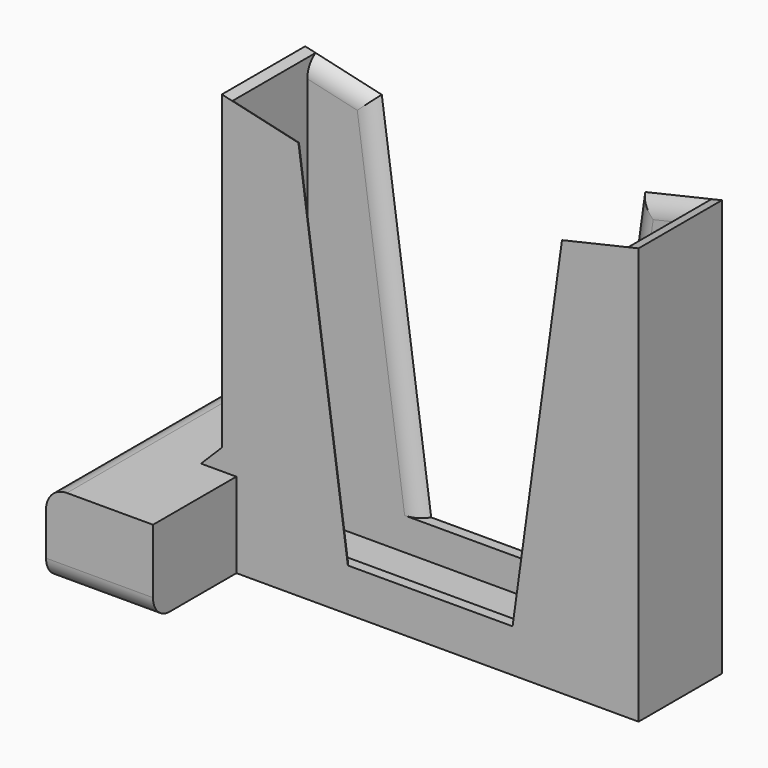
from build123d import *

# Parameters (mm, degrees)
F1_DEPTH     = 25.4
F2_T         = -2.54
F3_T4_DEPTH  = 109.6353324848
F3_T9_DEPTH  = 109.6353324848
F3_T14_DEPTH = 38.5537016023
F3_T19_DEPTH = 38.5537016023
F3_T24_DEPTH = 109.6353324848
F3_T29_DEPTH = 38.5537016023
F3_T34_DEPTH = 109.6353324848
F3_T39_DEPTH = 38.5537016023
F4_W         = 7.5721852481
F4_H         = 7.5721852481
F5_DEPTH     = 50.8
F6_SIZE      = 5.08
F7_R         = 5.08


# Not quite as in the source:
# - a fillet or chamfer that OpenCascade refuses, or shapes differently, is made with other operations: its cross-section is extruded or revolved along the edge and cut away or added


with BuildPart() as f1:
    # F0 (on Front) → F1 (new body)
    with BuildSketch(Plane.XZ):
        Polygon((-50.8, -50.8), (50.8, -50.8), (50.8, 50.8), (32.1275666356, 46.4897789061), (20.0797300786, -40.3164364398), (-20.0797300786, -40.3164364398), (-32.1275666356, 46.4897789061), (-50.8, 50.8), align=None)
    extrude(amount=F1_DEPTH)

    # F2
    f2_openings = [f1.faces().sort_by_distance(p)[0] for p in [
        (-41.463783, -12.7, 48.644889),
        (-26.103648, -12.7, 3.086671),
        (0, -12.7, -40.316436),
        (41.463783, -12.7, 48.644889),
        (26.103648, -12.7, 3.086671),
    ]]
    offset(amount=F2_T, openings=f2_openings)

    # F3: fillet of radius 5.08 on 8 edges, made by hand


with BuildPart() as f3_tool2:
    # F3_s3 → F3_t4 (new body)
    with BuildSketch(Plane(origin=(8.4495366949, 0, 60.8800010222), x_dir=(0, 1, 0), z_dir=(-0.1374722959, 0, -0.9905056122))):
        with BuildLine():
            ThreePointArc((0, 25.4314784161), (-1.8594090512, 27.2908874673), (-2.54, 29.8308874673))
            Line((-2.54, 29.8308874673), (-2.54, 25.4314784161))
            Line((-2.54, 25.4314784161), (0, 25.4314784161))
        make_face()
    extrude(amount=F3_T4_DEPTH)

    split(bisect_by=Plane.XY.offset(-40.3164364398), keep=Keep.TOP)


with BuildPart() as f1_1:
    add(f1.part)

    # F3_t1: cut F3_tool2
    add(f3_tool2.part, mode=Mode.SUBTRACT)


with BuildPart() as f3_tool7:
    # F3_s8 → F3_t9 (new body)
    with BuildSketch(Plane(origin=(6.6222841773, 0, -47.7144111022), x_dir=(0, 1, 0), z_dir=(-0.1374722959, 0, 0.9905056122))):
        with BuildLine():
            ThreePointArc((0, 25.4314784161), (-1.8594090512, 27.2908874673), (-2.54, 29.8308874673))
            Line((-2.54, 29.8308874673), (-2.54, 25.4314784161))
            Line((-2.54, 25.4314784161), (0, 25.4314784161))
        make_face()
    extrude(amount=F3_T9_DEPTH)

    split(bisect_by=Plane.XY.offset(-40.3164364398), keep=Keep.TOP)


with BuildPart() as f1_2:
    add(f1_1.part)

    # F3_t6: cut F3_tool7
    add(f3_tool7.part, mode=Mode.SUBTRACT)


with BuildPart() as f3_tool12:
    # F3_s13 → F3_t14 (new body)
    with BuildSketch(Plane(origin=(67.5399359806, 0, 15.5904723858), x_dir=(0, 1, 0), z_dir=(-0.9743774967, 0, -0.2249188607))):
        with BuildLine():
            ThreePointArc((0, -38.0724987065), (-1.8594090512, -36.2130896553), (-2.54, -33.6730896553))
            Line((-2.54, -33.6730896553), (-2.54, -38.0724987065))
            Line((-2.54, -38.0724987065), (0, -38.0724987065))
        make_face()
    extrude(amount=F3_T14_DEPTH)

    split(bisect_by=Plane.YZ.offset(48.26), keep=Keep.BOTTOM)


with BuildPart() as f1_3:
    add(f1_2.part)

    # F3_t11: cut F3_tool12
    add(f3_tool12.part, mode=Mode.SUBTRACT)


with BuildPart() as f3_tool17:
    # F3_s18 → F3_t19 (new body)
    with BuildSketch(Plane(origin=(-29.9740767247, 0, 6.9190177438), x_dir=(0, 1, 0), z_dir=(-0.9743774967, 0, 0.2249188607))):
        with BuildLine():
            ThreePointArc((0, -38.0724987065), (-1.8594090512, -36.2130896553), (-2.54, -33.6730896553))
            Line((-2.54, -33.6730896553), (-2.54, -38.0724987065))
            Line((-2.54, -38.0724987065), (0, -38.0724987065))
        make_face()
    extrude(amount=F3_T19_DEPTH)

    split(bisect_by=Plane.YZ.offset(-48.26), keep=Keep.TOP)


with BuildPart() as f1_4:
    add(f1_3.part)

    # F3_t16: cut F3_tool17
    add(f3_tool17.part, mode=Mode.SUBTRACT)


with BuildPart() as f3_tool22:
    # F3_s23 → F3_t24 (new body)
    with BuildSketch(Plane(origin=(6.6222841773, 0, -47.7144111022), x_dir=(0, 1, 0), z_dir=(-0.1374722959, 0, 0.9905056122))):
        with BuildLine():
            ThreePointArc((-25.4, 25.4314784161), (-23.5405909488, 27.2908874673), (-22.86, 29.8308874673))
            Line((-22.86, 29.8308874673), (-22.86, 25.4314784161))
            Line((-22.86, 25.4314784161), (-25.4, 25.4314784161))
        make_face()
    extrude(amount=F3_T24_DEPTH)

    split(bisect_by=Plane.XY.offset(-40.3164364398), keep=Keep.TOP)


with BuildPart() as f1_5:
    add(f1_4.part)

    # F3_t21: cut F3_tool22
    add(f3_tool22.part, mode=Mode.SUBTRACT)


with BuildPart() as f3_tool27:
    # F3_s28 → F3_t29 (new body)
    with BuildSketch(Plane(origin=(-29.9740767247, 0, 6.9190177438), x_dir=(0, 1, 0), z_dir=(-0.9743774967, 0, 0.2249188607))):
        with BuildLine():
            ThreePointArc((-25.4, -38.0724987065), (-23.5405909488, -36.2130896553), (-22.86, -33.6730896553))
            Line((-22.86, -33.6730896553), (-22.86, -38.0724987065))
            Line((-22.86, -38.0724987065), (-25.4, -38.0724987065))
        make_face()
    extrude(amount=F3_T29_DEPTH)

    split(bisect_by=Plane.YZ.offset(-48.26), keep=Keep.TOP)


with BuildPart() as f1_6:
    add(f1_5.part)

    # F3_t26: cut F3_tool27
    add(f3_tool27.part, mode=Mode.SUBTRACT)


with BuildPart() as f3_tool32:
    # F3_s33 → F3_t34 (new body)
    with BuildSketch(Plane(origin=(8.4495366949, 0, 60.8800010222), x_dir=(0, 1, 0), z_dir=(-0.1374722959, 0, -0.9905056122))):
        with BuildLine():
            ThreePointArc((-25.4, 25.4314784161), (-23.5405909488, 27.2908874673), (-22.86, 29.8308874673))
            Line((-22.86, 29.8308874673), (-22.86, 25.4314784161))
            Line((-22.86, 25.4314784161), (-25.4, 25.4314784161))
        make_face()
    extrude(amount=F3_T34_DEPTH)

    split(bisect_by=Plane.XY.offset(-40.3164364398), keep=Keep.TOP)


with BuildPart() as f1_7:
    add(f1_6.part)

    # F3_t31: cut F3_tool32
    add(f3_tool32.part, mode=Mode.SUBTRACT)


with BuildPart() as f3_tool37:
    # F3_s38 → F3_t39 (new body)
    with BuildSketch(Plane(origin=(67.5399359806, 0, 15.5904723858), x_dir=(0, 1, 0), z_dir=(-0.9743774967, 0, -0.2249188607))):
        with BuildLine():
            ThreePointArc((-25.4, -38.0724987065), (-23.5405909488, -36.2130896553), (-22.86, -33.6730896553))
            Line((-22.86, -33.6730896553), (-22.86, -38.0724987065))
            Line((-22.86, -38.0724987065), (-25.4, -38.0724987065))
        make_face()
    extrude(amount=F3_T39_DEPTH)

    split(bisect_by=Plane.YZ.offset(48.26), keep=Keep.BOTTOM)


with BuildPart() as f1_8:
    add(f1_7.part)

    # F3_t36: cut F3_tool37
    add(f3_tool37.part, mode=Mode.SUBTRACT)

    # F4 (on Front) → F5 (join)
    with BuildSketch(Plane.XZ):
        Polygon((-73.3337104321, -50.8196800947), (-54.8367798328, -50.8196800947), (-54.8367798328, -43.2474948466), (-47.2645945847, -43.2474948466), (-47.2645945847, -30.0912298262), (-73.3337104321, -30.0912298262), align=None)
        with Locations((-51.0506872088, -47.0335874707)):
            Rectangle(F4_W, F4_H)
    extrude(amount=F5_DEPTH)

    # F6
    f6_edges = [f1_8.edges().sort_by_distance(p)[0] for p in [
        (-50.8, -12.7, -30.09123),
    ]]
    chamfer(f6_edges, length=F6_SIZE)

    # F7
    f7_edges = [f1_8.edges().sort_by_distance(p)[0] for p in [
        (-73.33371, -25.4, -30.09123),
        (-60.299153, -50.8, -50.81968),
    ]]
    fillet(f7_edges, radius=F7_R)


solid = f1_8.part
